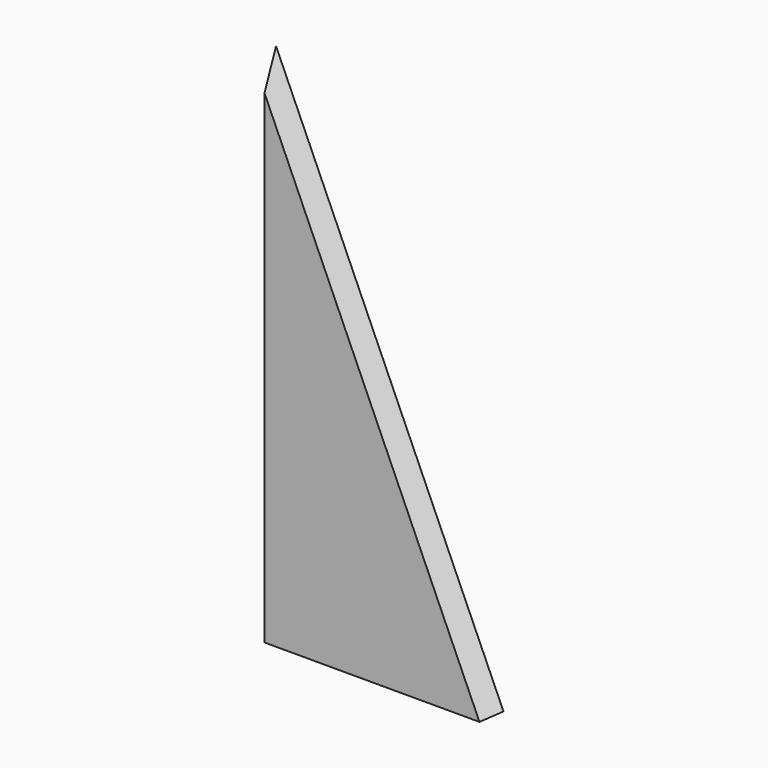
from build123d import *

# Parameters (mm, degrees)
F1_DEPTH = 19.05
F2_SIZE2 = 9.765156
F2_SIZE  = 19.04999
F3_SIZE2 = 19.04999
F3_SIZE  = 19.04999


# Not quite as in the source:
# - a fillet or chamfer is up to 0.001 mm smaller than in the source, because OpenCascade refuses the exact size


with BuildPart() as f1:
    # F0 (on Front) → F1 (new body)
    with BuildSketch(Plane.XZ):
        Polygon((-205.980393503, 296.4747510433), (-205.980393503, -389.3252489567), (98.819606497, -389.3252489567), align=None)
    extrude(amount=F1_DEPTH)

    # F2 (size 19.05 and 9.7651655461 in the source; OpenCascade refuses exactly that, so slightly less here)
    f2_edges = [f1.edges().sort_by_distance(p)[0] for p in [
        (-53.580394, 0, -389.325249),
    ]]
    f2_side = f1.faces().sort_by_distance((-53.580394, -9.525, -389.325249))[0]
    chamfer(f2_edges, length=F2_SIZE, length2=F2_SIZE2, reference=f2_side)

    # F3 (size 19.05 and 19.05 in the source; OpenCascade refuses exactly that, so slightly less here)
    f3_edges = [f1.edges().sort_by_distance(p)[0] for p in [
        (-53.580394, -19.05, -46.425249),
    ]]
    chamfer(f3_edges, length=F3_SIZE, length2=F3_SIZE2)


solid = f1.part
